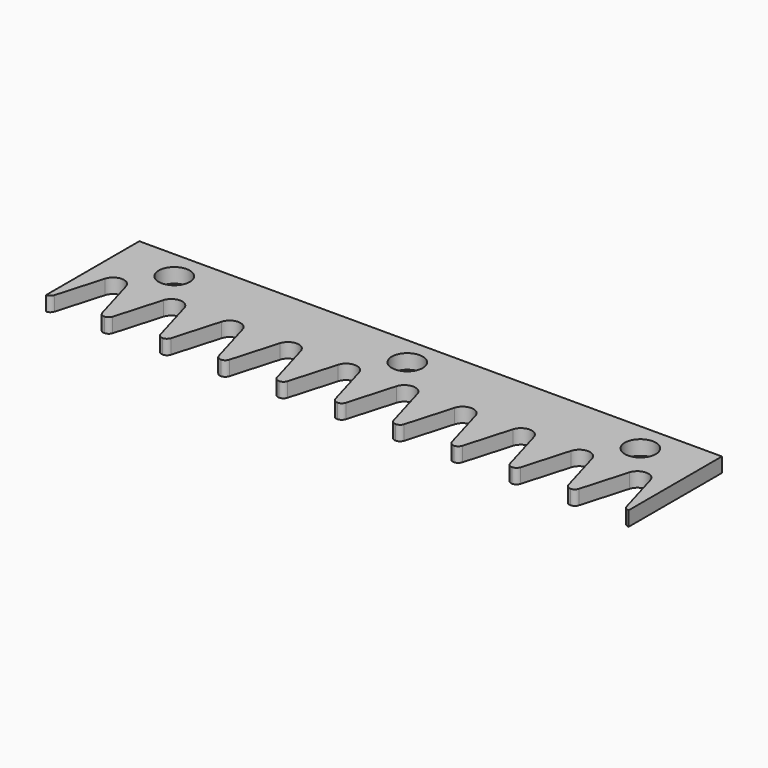
from build123d import *

# Parameters (mm, degrees)
F1_DEPTH = 3.175
F3_D     = 6.7564


# Not quite as in the source:
# - a feature names something its author has since deleted; it is built from what else it names


with BuildPart() as f1:
    # F0 (on Top) → F1 (new body)
    with BuildSketch(Plane.XY):
        with BuildLine():
            Line((0, 0), (0, 12.7))
            Line((0, 12.7), (-127, 12.7))
            Line((-127, 12.7), (-127, 0))
            Line((-127, 0), (-127, -12.7))
            ThreePointArc((-127, -12.7), (-126.2841905951, -12.4607975068), (-125.8560005402, -11.839303972))
            Line((-125.8560005402, -11.839303972), (-122.9379989196, -1.7213920559))
            ThreePointArc((-122.9379989196, -1.7213920559), (-120.65, 0), (-118.3620010804, -1.7213920559))
            Line((-118.3620010804, -1.7213920559), (-115.4439994598, -11.839303972))
            ThreePointArc((-115.4439994598, -11.839303972), (-115.0158094049, -12.4607975068), (-114.3, -12.7))
            ThreePointArc((-114.3, -12.7), (-113.5841905951, -12.4607975068), (-113.1560005402, -11.839303972))
            Line((-113.1560005402, -11.839303972), (-110.2379989196, -1.7213920559))
            ThreePointArc((-110.2379989196, -1.7213920559), (-107.95, 0), (-105.6620010804, -1.7213920559))
            Line((-105.6620010804, -1.7213920559), (-102.7439994598, -11.839303972))
            ThreePointArc((-102.7439994598, -11.839303972), (-102.3158094049, -12.4607975068), (-101.6, -12.7))
            ThreePointArc((-101.6, -12.7), (-100.8841905951, -12.4607975068), (-100.4560005402, -11.839303972))
            Line((-100.4560005402, -11.839303972), (-97.5379989196, -1.7213920559))
            ThreePointArc((-97.5379989196, -1.7213920559), (-95.25, 0), (-92.9620010804, -1.7213920559))
            Line((-92.9620010804, -1.7213920559), (-90.0439994598, -11.839303972))
            ThreePointArc((-90.0439994598, -11.839303972), (-89.6158094049, -12.4607975068), (-88.9, -12.7))
            ThreePointArc((-88.9, -12.7), (-88.1841905951, -12.4607975068), (-87.7560005402, -11.839303972))
            Line((-87.7560005402, -11.839303972), (-84.8379989196, -1.7213920559))
            ThreePointArc((-84.8379989196, -1.7213920559), (-82.55, 0), (-80.2620010804, -1.7213920559))
            Line((-80.2620010804, -1.7213920559), (-77.3439994598, -11.839303972))
            ThreePointArc((-77.3439994598, -11.839303972), (-76.9158094049, -12.4607975068), (-76.2, -12.7))
            ThreePointArc((-76.2, -12.7), (-75.4841905951, -12.4607975068), (-75.0560005402, -11.839303972))
            Line((-75.0560005402, -11.839303972), (-72.1379989196, -1.7213920559))
            ThreePointArc((-72.1379989196, -1.7213920559), (-69.85, 0), (-67.5620010804, -1.7213920559))
            Line((-67.5620010804, -1.7213920559), (-64.6439994598, -11.839303972))
            ThreePointArc((-64.6439994598, -11.839303972), (-64.2158094049, -12.4607975068), (-63.5, -12.7))
            ThreePointArc((-63.5, -12.7), (-62.7841905951, -12.4607975068), (-62.3560005402, -11.839303972))
            Line((-62.3560005402, -11.839303972), (-59.4379989196, -1.7213920559))
            ThreePointArc((-59.4379989196, -1.7213920559), (-57.15, 0), (-54.8620010804, -1.7213920559))
            Line((-54.8620010804, -1.7213920559), (-51.9439994598, -11.839303972))
            ThreePointArc((-51.9439994598, -11.839303972), (-51.5158094049, -12.4607975068), (-50.8, -12.7))
            ThreePointArc((-50.8, -12.7), (-50.0841905951, -12.4607975068), (-49.6560005402, -11.839303972))
            Line((-49.6560005402, -11.839303972), (-46.7379989196, -1.7213920559))
            ThreePointArc((-46.7379989196, -1.7213920559), (-44.45, 0), (-42.1620010804, -1.7213920559))
            Line((-42.1620010804, -1.7213920559), (-39.2439994598, -11.839303972))
            ThreePointArc((-39.2439994598, -11.839303972), (-38.8158094049, -12.4607975068), (-38.1, -12.7))
            ThreePointArc((-38.1, -12.7), (-37.3841905951, -12.4607975068), (-36.9560005402, -11.839303972))
            Line((-36.9560005402, -11.839303972), (-34.0379989196, -1.7213920559))
            ThreePointArc((-34.0379989196, -1.7213920559), (-31.75, 0), (-29.4620010804, -1.7213920559))
            Line((-29.4620010804, -1.7213920559), (-26.5439994598, -11.839303972))
            ThreePointArc((-26.5439994598, -11.839303972), (-26.1158094049, -12.4607975068), (-25.4, -12.7))
            ThreePointArc((-25.4, -12.7), (-24.6841905951, -12.4607975068), (-24.2560005402, -11.839303972))
            Line((-24.2560005402, -11.839303972), (-21.3379989196, -1.7213920559))
            ThreePointArc((-21.3379989196, -1.7213920559), (-19.05, 0), (-16.7620010804, -1.7213920559))
            Line((-16.7620010804, -1.7213920559), (-13.8439994598, -11.839303972))
            ThreePointArc((-13.8439994598, -11.839303972), (-13.4158094049, -12.4607975068), (-12.7, -12.7))
            ThreePointArc((-12.7, -12.7), (-11.9841905951, -12.4607975068), (-11.5560005402, -11.839303972))
            Line((-11.5560005402, -11.839303972), (-8.6379989196, -1.7213920559))
            ThreePointArc((-8.6379989196, -1.7213920559), (-6.35, 0), (-4.0620010804, -1.7213920559))
            Line((-4.0620010804, -1.7213920559), (-1.1439994598, -11.839303972))
            ThreePointArc((-1.1439994598, -11.839303972), (-0.7158094049, -12.4607975068), (0, -12.7))
            Line((0, -12.7), (0, 0))
        make_face()
    extrude(amount=F1_DEPTH)

    # F3 (through all)
    with Locations(Plane.XY.offset(3.175)):
        with Locations((-114.3, 6.35), (-63.5, 6.35), (-12.7, 6.35)):
            Hole(F3_D / 2)


solid = f1.part
